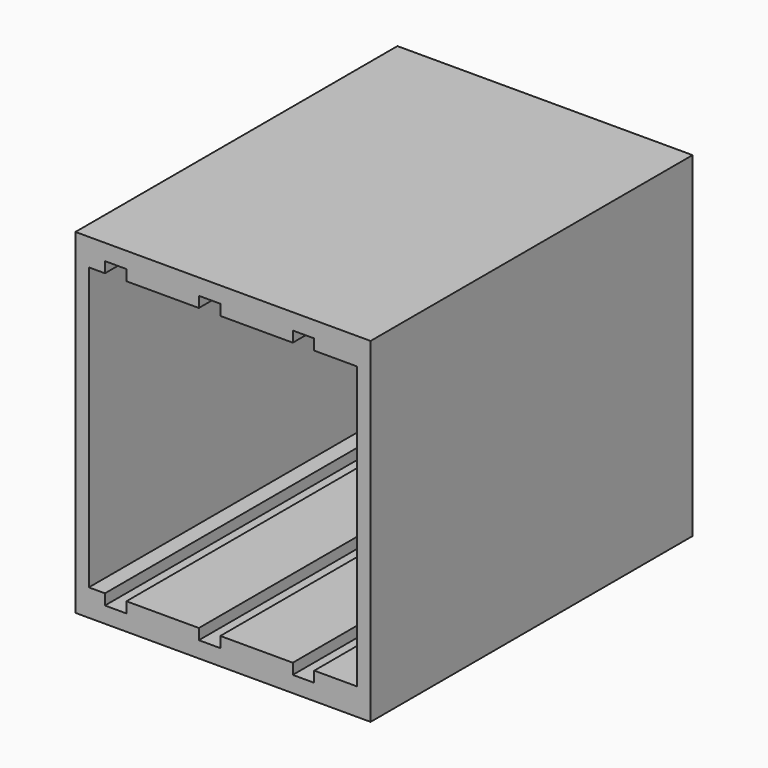
from build123d import *

# Parameters (mm, degrees)
F0_W     = 110
F0_H     = 125
F0_W_2   = 100
F0_H_2   = 105
F1_DEPTH = 150
F2_W     = 4
F2_H     = 4
F3_DEPTH = 150


# Not quite as in the source:
# - a pattern or mirror of a feature is missing from the dataset's text; its kind, count and spacing are read off the source's solid


with BuildPart() as f1:
    # F0 (on Front) → F1 (new body)
    with BuildSketch(Plane.XZ):
        Rectangle(F0_W, F0_H)
        Rectangle(F0_W_2, F0_H_2, mode=Mode.SUBTRACT)
    extrude(amount=F1_DEPTH)

    # F2 (on face) → F3 (cut, through all)
    with BuildSketch(Plane.XZ.offset(150)):
        with Locations((-42, 54.5)):
            Rectangle(F2_W, F2_H)
        with Locations((-38, 54.5)):
            Rectangle(F2_W, F2_H)
        with Locations((-3, 54.5)):
            Rectangle(F2_W, F2_H)
        with Locations((-7, 54.5)):
            Rectangle(F2_W, F2_H)
        with Locations((32, 54.5)):
            Rectangle(F2_W, F2_H)
        with Locations((28, 54.5)):
            Rectangle(F2_W, F2_H)
    f3 = extrude(amount=-F3_DEPTH, mode=Mode.SUBTRACT)

    # F3_copies: F3 across plane
    add(f3.mirror(Plane(origin=(0, 0, 0), x_dir=(-1, 0, 0), z_dir=(0, 0, -1))), mode=Mode.SUBTRACT)


solid = f1.part
